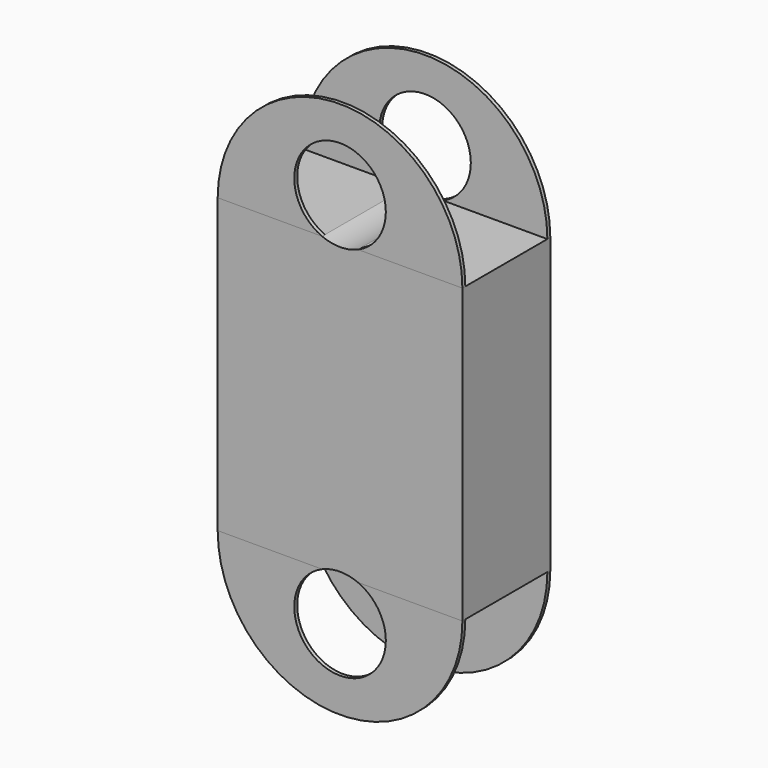
from build123d import *
from build123d import SkipClean  # not in build123d's __all__

# Parameters (mm, degrees)
F1_DEPTH = 19.05
F2_DEPTH = 0.635
F4_DEPTH = 0.635


with BuildPart() as f1:
    # F0 (on Front) → F1 (new body)
    with BuildSketch(Plane.XZ):
        with BuildLine():
            Line((7.6934193521, 67.6337401125), (-10.4047286745, 67.6337401125))
            Line((-10.4047286745, 67.6337401125), (-10.4047286745, 16.8337401125))
            Line((-10.4047286745, 16.8337401125), (7.6934193521, 16.8337401125))
            ThreePointArc((7.6934193521, 16.8337401125), (10.8042713255, 17.4687401125), (13.9151232988, 16.8337401125))
            Line((13.9151232988, 16.8337401125), (32.0132713255, 16.8337401125))
            Line((32.0132713255, 16.8337401125), (32.0132713255, 67.6337401125))
            Line((32.0132713255, 67.6337401125), (13.9151232988, 67.6337401125))
            ThreePointArc((13.9151232988, 67.6337401125), (10.8042713255, 66.9987401125), (7.6934193521, 67.6337401125))
        make_face()
    extrude(amount=F1_DEPTH)

    # F0 (on Front) → F2 (join)
    with BuildSketch(Plane.XZ):
        with BuildLine():
            ThreePointArc((32.0132713255, 67.6337401125), (10.8042713255, 88.8427401125), (-10.4047286745, 67.6337401125))
            Line((-10.4047286745, 67.6337401125), (7.6934193521, 67.6337401125))
            ThreePointArc((7.6934193521, 67.6337401125), (6.4275420266, 81.5580334417), (18.7417713255, 74.9362401125))
            ThreePointArc((18.7417713255, 74.9362401125), (17.4260646546, 70.5595108136), (13.9151232988, 67.6337401125))
            Line((13.9151232988, 67.6337401125), (32.0132713255, 67.6337401125))
        make_face()
        with BuildLine():
            Line((7.6934193521, 67.6337401125), (-10.4047286745, 67.6337401125))
            Line((-10.4047286745, 67.6337401125), (-10.4047286745, 16.8337401125))
            Line((-10.4047286745, 16.8337401125), (7.6934193521, 16.8337401125))
            ThreePointArc((7.6934193521, 16.8337401125), (10.8042713255, 17.4687401125), (13.9151232988, 16.8337401125))
            Line((13.9151232988, 16.8337401125), (32.0132713255, 16.8337401125))
            Line((32.0132713255, 16.8337401125), (32.0132713255, 67.6337401125))
            Line((32.0132713255, 67.6337401125), (13.9151232988, 67.6337401125))
            ThreePointArc((13.9151232988, 67.6337401125), (10.8042713255, 66.9987401125), (7.6934193521, 67.6337401125))
        make_face()
        with BuildLine():
            Line((7.6934193521, 16.8337401125), (-10.4047286745, 16.8337401125))
            ThreePointArc((-10.4047286745, 16.8337401125), (10.8042713255, -4.3752598875), (32.0132713255, 16.8337401125))
            Line((32.0132713255, 16.8337401125), (13.9151232988, 16.8337401125))
            ThreePointArc((13.9151232988, 16.8337401125), (17.4260646546, 13.9079694114), (18.7417713255, 9.5312401125))
            ThreePointArc((18.7417713255, 9.5312401125), (6.4275420266, 2.9094467834), (7.6934193521, 16.8337401125))
        make_face()
    extrude(amount=F2_DEPTH)

    # F3 (on face) → F4 (join)
    with BuildSketch(Plane.XZ.offset(19.05)):
        with BuildLine():
            ThreePointArc((-10.4047286745, 16.8337401125), (10.8042713255, -4.3752598875), (32.0132713255, 16.8337401125))
            Line((32.0132713255, 16.8337401125), (13.9151232988, 16.8337401125))
            ThreePointArc((13.9151232988, 16.8337401125), (17.4260646546, 13.9079694114), (18.7417713255, 9.5312401125))
            ThreePointArc((18.7417713255, 9.5312401125), (6.4275420266, 2.9094467834), (7.6934193521, 16.8337401125))
            Line((7.6934193521, 16.8337401125), (-10.4047286745, 16.8337401125))
        make_face()
        with BuildLine():
            Line((13.9151232988, 67.6337401125), (32.0132713255, 67.6337401125))
            ThreePointArc((32.0132713255, 67.6337401125), (10.8042713255, 88.8427401125), (-10.4047286745, 67.6337401125))
            Line((-10.4047286745, 67.6337401125), (7.6934193521, 67.6337401125))
            ThreePointArc((7.6934193521, 67.6337401125), (6.4275420266, 81.5580334417), (18.7417713255, 74.9362401125))
            ThreePointArc((18.7417713255, 74.9362401125), (17.4260646546, 70.5595108136), (13.9151232988, 67.6337401125))
        make_face()
    with SkipClean():  # cleaning this boolean's faces spoils the solid; the shape is the same uncleaned
        extrude(amount=-F4_DEPTH)


solid = f1.part
